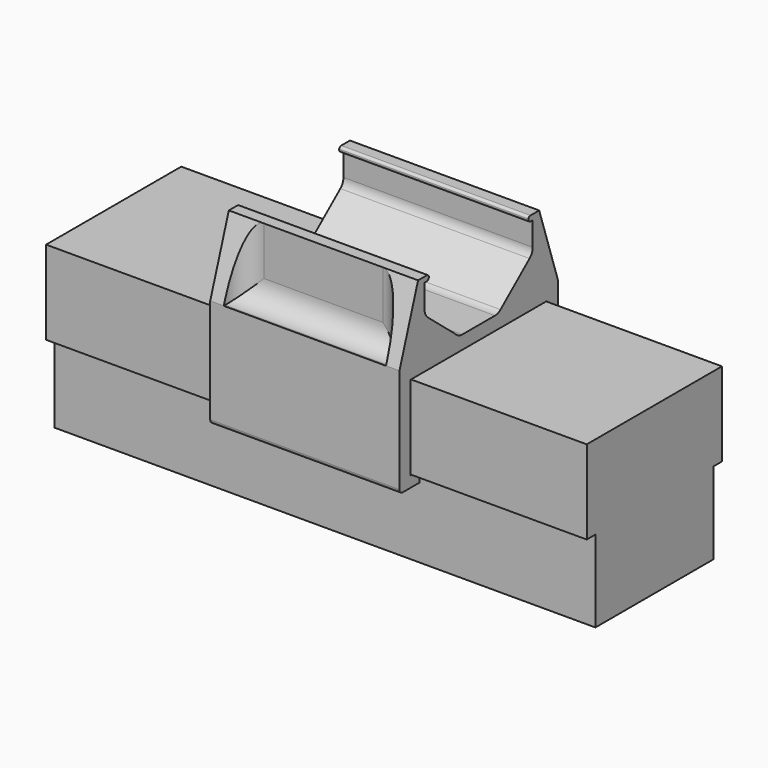
from build123d import *

# Parameters (mm, degrees)
F0_W      = 54.5
F0_H      = 30.2627416849
F1_DEPTH  = 100
F2_W      = 5
F2_H      = 4
F3_DEPTH  = 35
F5_DEPTH  = 70
F8_DEPTH  = 5
F10_DEPTH = 5
F11_R     = 8
F12_R     = 1.5


with BuildPart() as f1:
    # F0 (on Right) → F1 (new body, symmetric)
    with BuildSketch(Plane.YZ):
        Polygon((31.25, 0), (-31.25, 0), (-31.25, -31), (-27.25, -31), (27.25, -31), (31.25, -31), align=None)
        with Locations((0, -46.1313708425)):
            Rectangle(F0_W, F0_H)
    extrude(amount=F1_DEPTH, both=True)


with BuildPart() as f3:
    # F2 (on Right) → F3 (new body, symmetric)
    with BuildSketch(Plane.YZ):
        Polygon((0, 5), (0, 0), (31.6, 0), (31.6, -31.2), (29.1, -31.2), (29.1, -35.2), (36.6, -35.2), (36.6, 5), align=None)
        Polygon((-31.6, 0), (0, 0), (0, 5), (-36.6, 5), (-36.6, -35.2), (-29.1, -35.2), (-29.1, -31.2), (-31.6, -31.2), align=None)
        with Locations((-26.6, -33.2)):
            Rectangle(F2_W, F2_H)
    extrude(amount=F3_DEPTH, both=True)

    # F4 (on face) → F5 (join, through all)
    with BuildSketch(Plane.YZ.offset(35)):
        with BuildLine():
            Line((-28, 5), (-7.5545838353, 5))
            ThreePointArc((-7.5545838353, 5), (-8.9139701192, 5.238076432), (-10.1115374849, 5.9239655343))
            Line((-10.1115374849, 5.9239655343), (-23.5569536496, 17.1004677212))
            ThreePointArc((-23.5569536496, 17.1004677212), (-24.6213129248, 18.4776517812), (-25, 20.1765021869))
            Line((-25, 20.1765021869), (-25, 29))
            Line((-25, 29), (-24, 29))
            ThreePointArc((-24, 29), (-23.227192279, 29.3653597662), (-23.0190902545, 30.1944635473))
            ThreePointArc((-23.0190902545, 30.1944635473), (-23.3738776782, 30.7398834056), (-23.9891411693, 30.9515618745))
            Line((-23.9891411693, 30.9515618745), (-28, 30.9515618745))
            Line((-28, 30.9515618745), (-28, 5))
        make_face()
        with BuildLine():
            Line((25, 5), (25, 20.1765021869))
            ThreePointArc((25, 20.1765021869), (24.6213129248, 18.4776517812), (23.5569536496, 17.1004677212))
            Line((23.5569536496, 17.1004677212), (10.1115374849, 5.9239655343))
            ThreePointArc((10.1115374849, 5.9239655343), (8.9139701192, 5.238076432), (7.5545838353, 5))
            Line((7.5545838353, 5), (25, 5))
        make_face()
        with BuildLine():
            Line((24, 29), (25, 29))
            Line((25, 29), (25, 20.1765021869))
            Line((25, 20.1765021869), (25, 5))
            Line((25, 5), (28, 5))
            Line((28, 5), (28, 30.9515618745))
            Line((28, 30.9515618745), (23.9891411693, 30.9515618745))
            ThreePointArc((23.9891411693, 30.9515618745), (23.3738776782, 30.7398834056), (23.0190902545, 30.1944635473))
            ThreePointArc((23.0190902545, 30.1944635473), (23.227192279, 29.3653597662), (24, 29))
        make_face()
    extrude(amount=-F5_DEPTH)

    # F6: union 

    # F7 (on face) → F8 (join)
    with BuildSketch(Plane.YZ.offset(35)):
        Polygon((28, 30.9515618745), (28, 5), (36.6, 5), align=None)
        Polygon((-28, 30.9515618745), (-36.6, 5), (-28, 5), align=None)
    extrude(amount=-F8_DEPTH)

    # F9 (on face) → F10 (join)
    with BuildSketch(Plane(origin=(-35, 0, 0), x_dir=(0, -1, 0), z_dir=(-1, 0, 0))):
        Polygon((-28, 30.9515618745), (-36.6, 5), (-28, 5), align=None)
        Polygon((36.6, 5), (28, 30.9515618745), (28, 5), align=None)
    extrude(amount=-F10_DEPTH)

    # F11
    f11_edges = [f3.edges().sort_by_distance(p)[0] for p in [
        (0, 28, 5),
        (30, -28, 17.975781),
        (-30, -28, 17.975781),
        (30, 28, 17.975781),
        (-30, 28, 17.975781),
        (0, -28, 5),
    ]]
    fillet(f11_edges, radius=F11_R)

    # F12
    f12_edges = [f3.edges().sort_by_distance(p)[0] for p in [
        (0, -36.6, -35.2),
        (0, 36.6, -35.2),
        (0, 29.1, -35.2),
        (0, -24.1, -35.2),
    ]]
    fillet(f12_edges, radius=F12_R)


solid = Compound([f1.part, f3.part])
